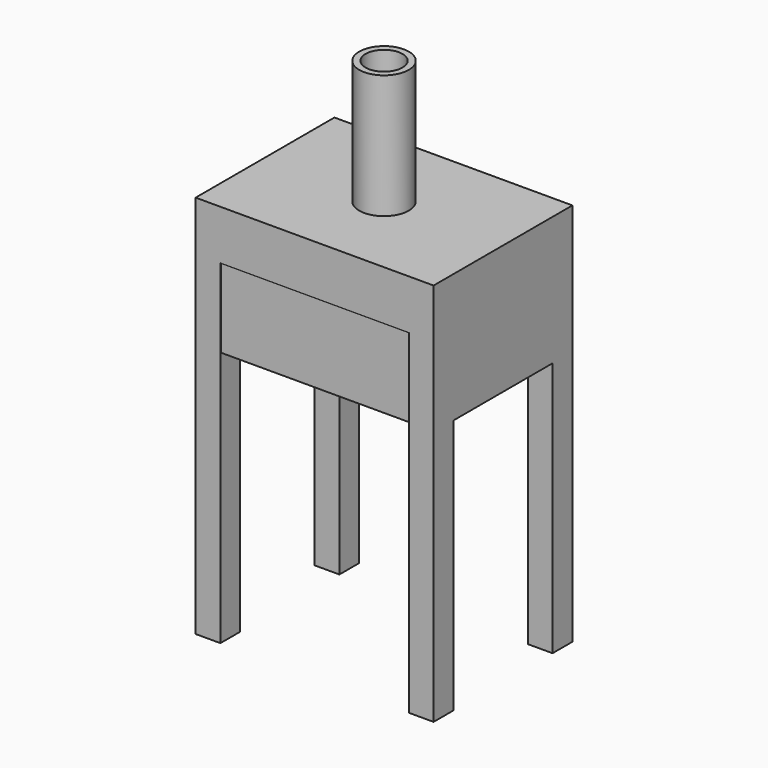
from build123d import *

# Parameters (mm, degrees)
F0_W      = 480
F0_H      = 350
F1_DEPTH  = 100
F2_W      = 50
F2_H      = 50
F3_DEPTH  = 675
F4_W      = 50
F4_H      = 50
F5_DEPTH  = 675
F6_W      = 50
F6_H      = 50
F7_DEPTH  = 675
F8_W      = 50
F8_H      = 50
F9_DEPTH  = 675
F10_R     = 50
F10_R_2   = 37.3037381585
F11_DEPTH = 250
F14_W     = 430
F14_H     = 139.1179516912
F15_DEPTH = 160
F16_DEPTH = 209
F17_W     = 49.8938559854
F17_H     = 160
F18_DEPTH = 430


# Not quite as in the source:
# - a feature names something its author has since deleted; it is built from what else it names
# - the program builds the solid bodies; features that only make, move or delete a surface that nothing else refers to are left out


with BuildPart() as f1:
    # F0 (on Top) → F1 (new body)
    with BuildSketch(Plane.XY):
        Rectangle(F0_W, F0_H)
    extrude(amount=F1_DEPTH)

    # F2 (on face) → F3 (join)
    with BuildSketch(Plane(origin=(0, 0, 0), x_dir=(1, 0, 0), z_dir=(0, 0, -1))):
        with Locations((215, 150)):
            Rectangle(F2_W, F2_H)
    extrude(amount=F3_DEPTH)

    # F4 (on face) → F5 (join)
    with BuildSketch(Plane(origin=(0, 0, 0), x_dir=(1, 0, 0), z_dir=(0, 0, -1))):
        with Locations((215, -150)):
            Rectangle(F4_W, F4_H)
    extrude(amount=F5_DEPTH)

    # F6 (on face) → F7 (join)
    with BuildSketch(Plane(origin=(0, 0, 0), x_dir=(1, 0, 0), z_dir=(0, 0, -1))):
        with Locations((-215, -150)):
            Rectangle(F6_W, F6_H)
    extrude(amount=F7_DEPTH)

    # F8 (on face) → F9 (join)
    with BuildSketch(Plane(origin=(0, 0, 0), x_dir=(1, 0, 0), z_dir=(0, 0, -1))):
        with Locations((-215, 150)):
            Rectangle(F8_W, F8_H)
    extrude(amount=F9_DEPTH)

    # F10 (on face) → F11 (join)
    with BuildSketch(Plane.XY.offset(100)):
        Circle(F10_R)
        Circle(F10_R_2, mode=Mode.SUBTRACT)
    extrude(amount=F11_DEPTH)

    # F14 (on face) → F15 (join)
    with BuildSketch(Plane(origin=(0, 0, 0), x_dir=(1, 0, 0), z_dir=(0, 0, -1))):
        with Locations((25, -105.4410241544)):
            Rectangle(F14_W, F14_H)
    extrude(amount=F15_DEPTH)

    # F16 (add): a face of the model
    f16_faces = [f1.faces().sort_by_distance(p)[0] for p in [
        (25, 35.8820483088, -80),
    ]]
    extrude(f16_faces, amount=F16_DEPTH)

    # F17 (on face) → F18 (join)
    with BuildSketch(Plane(origin=(-190, 0, 0), x_dir=(0, -1, 0), z_dir=(-1, 0, 0))):
        with Locations((-149.9469279927, -80)):
            Rectangle(F17_W, F17_H)
    extrude(amount=-F18_DEPTH)


solid = f1.part
